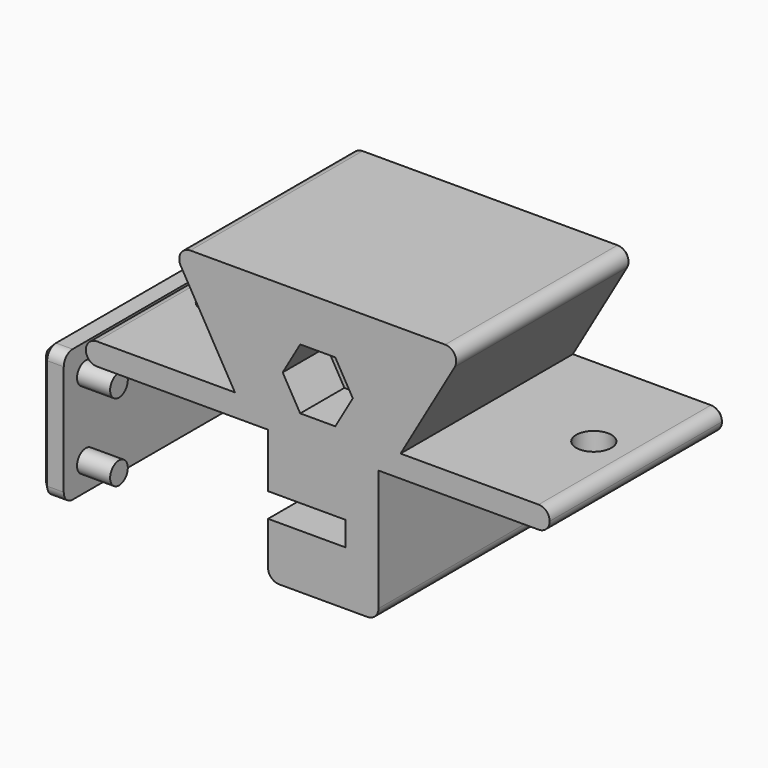
from build123d import *

# Parameters (mm, degrees)
F0_W       = 10
F0_H       = 12
F1_DEPTH   = 20
F2_R       = 2.5
F2_R_2     = 1.15
F3_DEPTH   = 7
F4_R       = 1.25
F5_DEPTH   = 25.501
F7_DEPTH   = 1
F8_W       = 6
F8_H       = 5
F9_DEPTH   = 2
F11_W      = 20
F11_H      = 12
F11_R      = 1.75
F12_DEPTH  = 2
F13_R      = 1
F14_DEPTH  = 3
F15_R      = 1.6
F16_DEPTH  = 14.001
F18_DEPTH  = 5
F19_R      = 1.6
F20_DEPTH  = 15.001
F21_R      = 0.99999
F21_2_R    = 0.99999
F22_SIZE   = 0.5
F22_2_SIZE = 0.5


# Not quite as in the source:
# - a fillet or chamfer is up to 0.001 mm smaller than in the source, because OpenCascade refuses the exact size


with BuildPart() as f1:
    # F0 (on Front) → F1 (new body)
    with BuildSketch(Plane.XZ):
        with BuildLine():
            Line((-12.4074772881, 9.5), (-7.5, 1))
            Line((-7.5, 1), (7.5, 1))
            Line((7.5, 1), (12.4074772881, 9.5))
            ThreePointArc((12.4074772881, 9.5), (12.4074772881, 10.5), (11.5414518843, 11))
            Line((11.5414518843, 11), (-11.5414518843, 11))
            ThreePointArc((-11.5414518843, 11), (-12.4074772881, 10.5), (-12.4074772881, 9.5))
        make_face()
        Polygon((7.5, 1), (-7.5, 1), (-21, 1), (-21, -1), (-4.5, -1), (5.5, -1), (21, -1), (21, 1), align=None)
        with Locations((0.5, -7)):
            Rectangle(F0_W, F0_H)
    extrude(amount=F1_DEPTH)

    # F2 (on face) → F3 (cut)
    with BuildSketch(Plane(origin=(-4.5, 0, 0), x_dir=(0, -1, 0), z_dir=(-1, 0, 0))):
        with BuildLine():
            ThreePointArc((9.8457769046, -8.1), (9.9612565947, -7.5553793215), (10, -7))
            ThreePointArc((10, -7), (9.9612565947, -6.4446206785), (9.8457769046, -5.9))
            Line((9.8457769046, -5.9), (9.8457769046, -8.1))
        make_face()
        with BuildLine():
            ThreePointArc((9.8457769046, -5.9), (9.9612565947, -6.4446206785), (10, -7))
            ThreePointArc((10, -7), (9.9612565947, -7.5553793215), (9.8457769046, -8.1))
            Line((9.8457769046, -8.1), (20, -8.1))
            Line((20, -8.1), (20, -5.9))
            Line((20, -5.9), (9.8457769046, -5.9))
        make_face()
        with BuildLine():
            Line((9.8457769046, -8.1), (9.8457769046, -5.9))
            ThreePointArc((9.8457769046, -5.9), (2, -7), (9.8457769046, -8.1))
        make_face()
        with Locations((6, -7)):
            Circle(F2_R, mode=Mode.SUBTRACT)
        with Locations((17.5, -10.5)):
            Circle(F2_R_2)
        with Locations((17.5, -3.5)):
            Circle(F2_R_2)
    extrude(amount=-F3_DEPTH, mode=Mode.SUBTRACT)

    # F4 (on face) → F5 (cut, through all)
    with BuildSketch(Plane(origin=(-4.5, 0, 0), x_dir=(0, -1, 0), z_dir=(-1, 0, 0))):
        with Locations((6, -7)):
            Circle(F4_R)
    extrude(amount=-F5_DEPTH, mode=Mode.SUBTRACT)

    # F6 (on face) → F7 (join)
    with BuildSketch(Plane(origin=(-4.5, 0, 0), x_dir=(0, -1, 0), z_dir=(-1, 0, 0))):
        with BuildLine():
            Line((6, -5.1), (6, -4.5))
            ThreePointArc((6, -4.5), (3.5, -7), (6, -9.5))
            Line((6, -9.5), (6, -8.9))
            ThreePointArc((6, -8.9), (4.1, -7), (6, -5.1))
        make_face()
    extrude(amount=F7_DEPTH)

    # F8 (on face) → F9 (join)
    with BuildSketch(Plane(origin=(-5.5, 0, 0), x_dir=(0, -1, 0), z_dir=(-1, 0, 0))):
        with Locations((3, -7)):
            Rectangle(F8_W, F8_H)
    extrude(amount=F9_DEPTH)

    # F15 (on face) → F16 (cut, through all)
    with BuildSketch(Plane.XY.offset(1)):
        with Locations((17, -10)):
            Circle(F15_R)
        with Locations((-17, -10)):
            Circle(F15_R)
    extrude(amount=-F16_DEPTH, mode=Mode.SUBTRACT)

    # F17 (on face) → F18 (cut)
    with BuildSketch(Plane.XZ.offset(20)):
        Polygon((-1.5877132403, 1.25), (1.5877132403, 1.25), (3.1754264805, 4), (1.5877132403, 6.75), (-1.5877132403, 6.75), (-3.1754264805, 4), align=None)
    extrude(amount=-F18_DEPTH, mode=Mode.SUBTRACT)

    # F19 (on face) → F20 (cut, through all)
    with BuildSketch(Plane.XZ.offset(15)):
        with Locations((0, 4)):
            Circle(F19_R)
    extrude(amount=-F20_DEPTH, mode=Mode.SUBTRACT)

    # F21 (radius 1 in the source; OpenCascade refuses exactly that, so slightly less here)
    f21_edges = [f1.edges().sort_by_distance(p)[0] for p in [
        (5.5, -10, -13),
        (21, -10, -1),
        (21, -10, 1),
        (-21, -10, -1),
        (-21, -10, 1),
        (-4.5, -10, -13),
    ]]
    fillet(f21_edges, radius=F21_R)

    # F22
    f22_edges = [f1.edges().sort_by_distance(p)[0] for p in [
        (-4.5, 0, -6.500005),
        (-12.250005, 0, -1),
        (-9.953739, 0, 5.25),
        (12.750005, 0, -1),
    ]]
    chamfer(f22_edges, length=F22_SIZE)


with BuildPart() as f12:
    # F11 (on offset) → F12 (new body)
    with BuildSketch(Plane.YZ.offset(-25)):
        with Locations((-10, -7)):
            Rectangle(F11_W, F11_H)
        with Locations((-6, -7)):
            Circle(F11_R, mode=Mode.SUBTRACT)
    extrude(amount=F12_DEPTH)

    # F13 (on face) → F14 (join)
    with BuildSketch(Plane.YZ.offset(-23)):
        with Locations((-17.5, -10.5)):
            Circle(F13_R)
        with Locations((-17.5, -3.5)):
            Circle(F13_R)
    extrude(amount=F14_DEPTH)

    # F21#2 (radius 1 in the source; OpenCascade refuses exactly that, so slightly less here)
    f21_2_edges = [f12.edges().sort_by_distance(p)[0] for p in [
        (-24, -20, -1),
        (-24, 0, -1),
        (-24, -20, -13),
        (-24, 0, -13),
    ]]
    fillet(f21_2_edges, radius=F21_2_R)

    # F22#2
    f22_2_edges = [f12.edges().sort_by_distance(p)[0] for p in [
        (-25, -10, -1),
    ]]
    chamfer(f22_2_edges, length=F22_2_SIZE)


solid = Compound([f1.part, f12.part])
